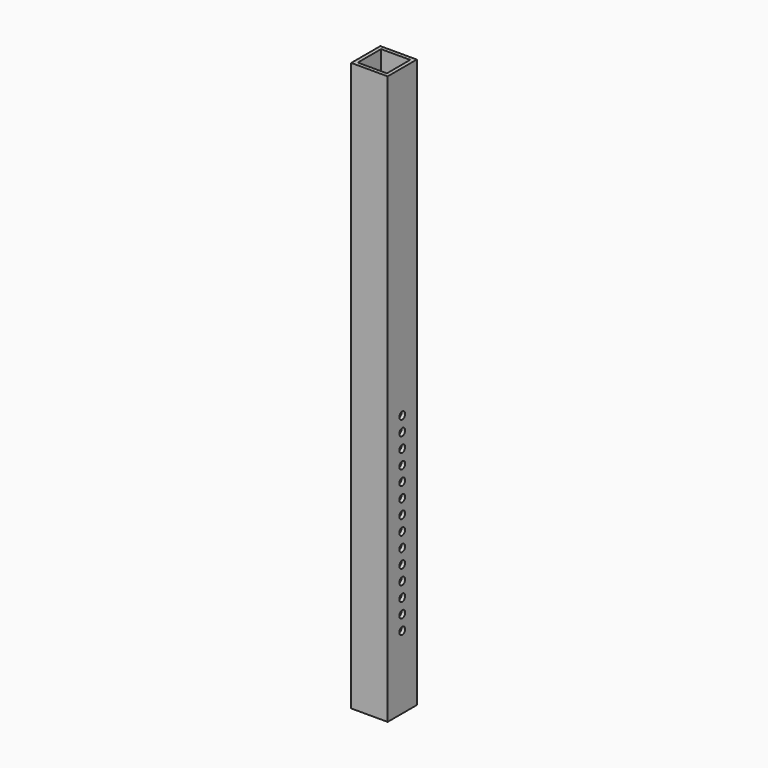
from build123d import *

# Parameters (mm, degrees)
F0_W     = 63.5
F0_H     = 63.5
F0_W_2   = 50.8
F0_H_2   = 50.8
F1_DEPTH = 990.6
F3_D     = 12.7


# Not quite as in the source:
# - a length typed as a fraction of an inch, garbled in the dataset ("3 / 203.2 mm" for 3/8 in), is restored


with BuildPart() as f1:
    # F0 (on Top) → F1 (new body)
    with BuildSketch(Plane.XY):
        Rectangle(F0_W, F0_H)
        Rectangle(F0_W_2, F0_H_2, mode=Mode.SUBTRACT)
    extrude(amount=F1_DEPTH)

    # F3 (through all)
    with Locations(Plane.YZ.offset(31.75)):
        with Locations((0, 127), (0, 152.4), (0, 177.8), (0, 203.2), (0, 228.6), (0, 254), (0, 279.4), (0, 304.8), (0, 330.2), (0, 355.6), (0, 381), (0, 406.4), (0, 431.8), (0, 457.2)):
            Hole(F3_D / 2)


solid = f1.part
